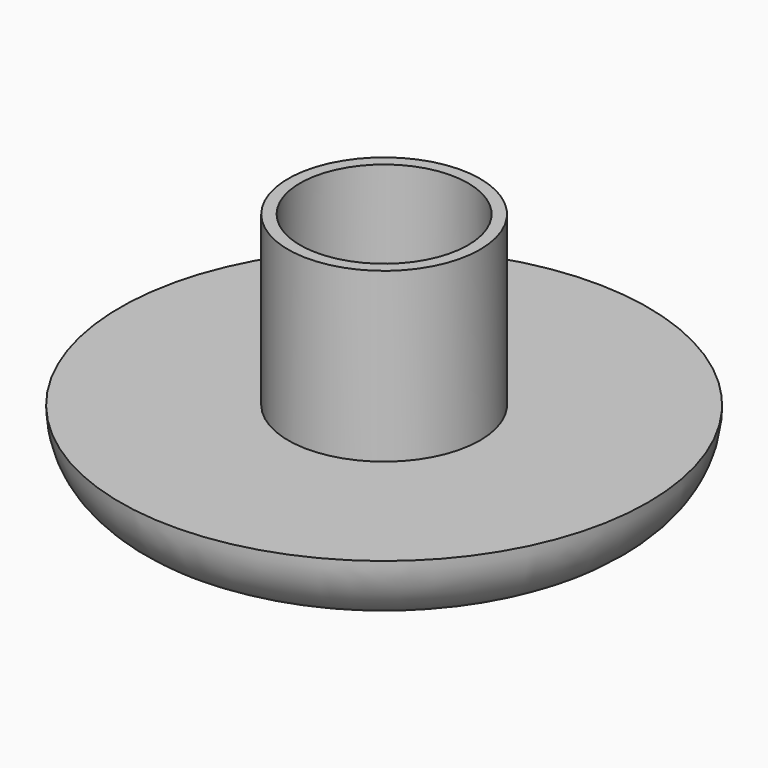
from build123d import *

# Parameters (mm, degrees)
F0_R     = 11
F1_DEPTH = 3
F2_R     = 4
F2_R_2   = 3.5
F3_DEPTH = 7
F4_R     = 2.99999


# Not quite as in the source:
# - a fillet or chamfer is up to 0.001 mm smaller than in the source, because OpenCascade refuses the exact size


with BuildPart() as f1:
    # F0 (on Top) → F1 (new body)
    with BuildSketch(Plane.XY):
        Circle(F0_R)
    extrude(amount=F1_DEPTH)

    # F2 (on face) → F3 (join)
    with BuildSketch(Plane.XY.offset(3)):
        Circle(F2_R)
        Circle(F2_R_2, mode=Mode.SUBTRACT)
    extrude(amount=F3_DEPTH)

    # F4 (radius 3 in the source; OpenCascade refuses exactly that, so slightly less here)
    f4_edges = [f1.edges().sort_by_distance(p)[0] for p in [
        (-11, 0, 0),
    ]]
    fillet(f4_edges, radius=F4_R)


solid = f1.part
